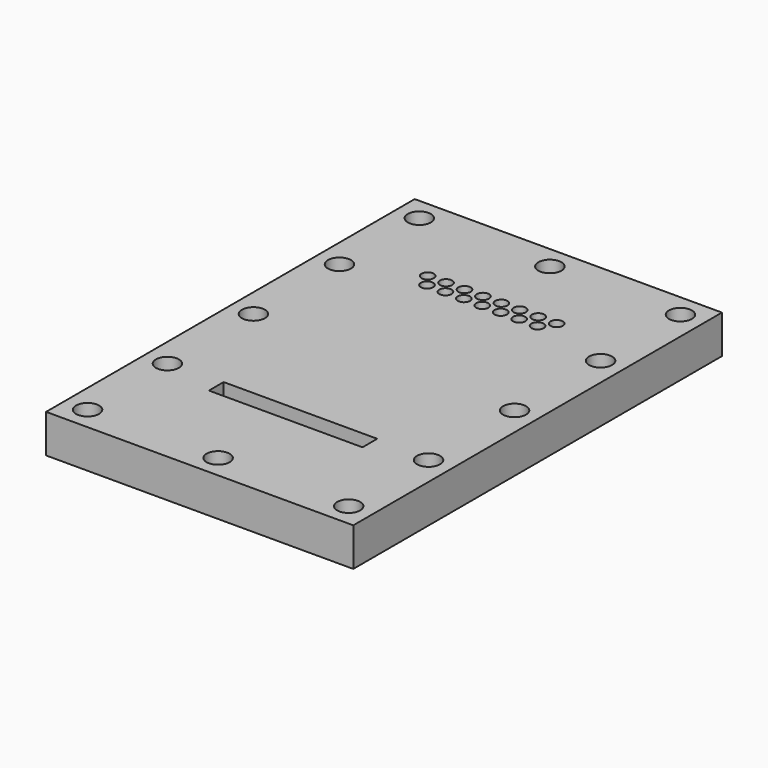
from build123d import *

# Parameters (mm, degrees)
F0_W     = 100
F0_H     = 150
F1_DEPTH = 12.5
F2_R     = 3.75
F3_DEPTH = 25
F4_W     = 50
F4_H     = 6
F5_DEPTH = 25
F6_R     = 2
F7_DEPTH = 25


# Not quite as in the source:
# - a feature names something its author has since deleted; it is built from what else it names


with BuildPart() as f1:
    # F0 (on Top) → F1 (new body)
    with BuildSketch(Plane.XY):
        Rectangle(F0_W, F0_H)
    extrude(amount=F1_DEPTH)

    # F2 (on face) → F3 (cut)
    with BuildSketch(Plane.XY.offset(12.5)):
        with Locations((-42.5, 67.5)):
            Circle(F2_R)
        with Locations((-42.5, 0)):
            Circle(F2_R)
        with Locations((-42.5, -35)):
            Circle(F2_R)
        with Locations((-42.5, -67.5)):
            Circle(F2_R)
        with Locations((0, -67.5)):
            Circle(F2_R)
        with Locations((-42.5, 35)):
            Circle(F2_R)
        with Locations((42.5, -67.5)):
            Circle(F2_R)
        with Locations((42.5, -35)):
            Circle(F2_R)
        with Locations((42.5, 0)):
            Circle(F2_R)
        with Locations((42.5, 35)):
            Circle(F2_R)
        with Locations((42.5, 67.5)):
            Circle(F2_R)
        with Locations((0, 67.5)):
            Circle(F2_R)
    extrude(amount=-F3_DEPTH, mode=Mode.SUBTRACT)

    # F4 (on face) → F5 (cut)
    with BuildSketch(Plane.XY.offset(12.5)):
        with Locations((0, -37)):
            Rectangle(F4_W, F4_H)
    extrude(amount=-F5_DEPTH, mode=Mode.SUBTRACT)

    # F6 (on face) → F7 (cut)
    with BuildSketch(Plane.XY.offset(12.5)):
        with Locations((-18, 40)):
            Circle(F6_R)
        with Locations((-15, 44)):
            Circle(F6_R)
        with Locations((-12, 40)):
            Circle(F6_R)
        with Locations((-9, 44)):
            Circle(F6_R)
        with Locations((-6, 40)):
            Circle(F6_R)
        with Locations((0, 40)):
            Circle(F6_R)
        with Locations((-3, 44)):
            Circle(F6_R)
        with Locations((-21, 44)):
            Circle(F6_R)
        with Locations((15, 44)):
            Circle(F6_R)
        with Locations((6, 40)):
            Circle(F6_R)
        with Locations((18, 40)):
            Circle(F6_R)
        with Locations((3, 44)):
            Circle(F6_R)
        with Locations((21, 44)):
            Circle(F6_R)
        with Locations((12, 40)):
            Circle(F6_R)
        with Locations((9, 44)):
            Circle(F6_R)
    extrude(amount=-F7_DEPTH, mode=Mode.SUBTRACT)


solid = f1.part
